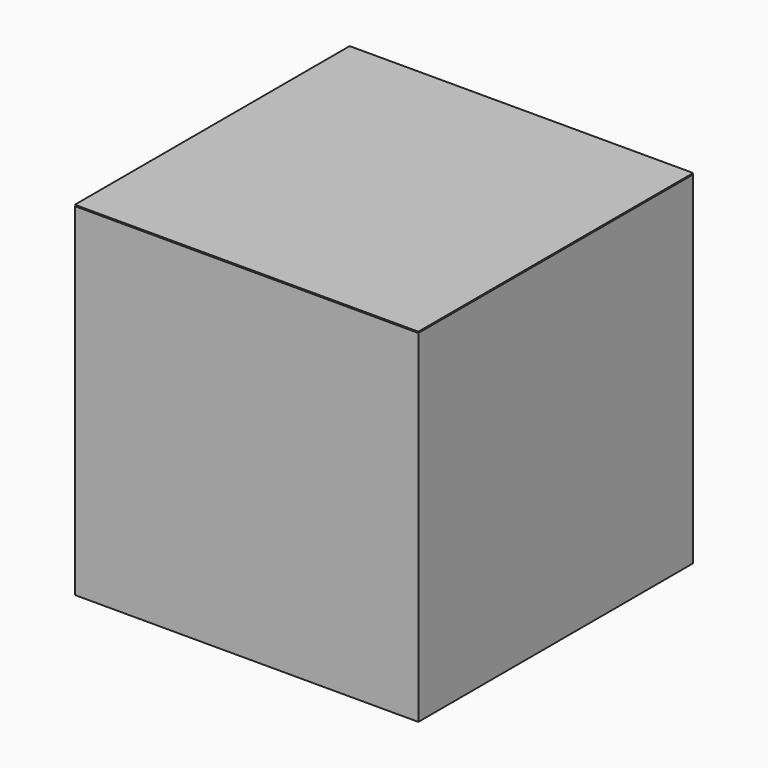
from build123d import *

# Parameters (mm, degrees)
F0_W         = 70
F0_H         = 70
F1_DEPTH     = 35
F2_T         = -3
F3_W         = 70
F3_H         = 70
F4_DEPTH     = 3
F5_SIZE      = 2.99999
F6_T1_DEPTH  = 64
F6_T3_DEPTH  = 64
F6_T9_DEPTH  = 72.3579697109
F6_T15_DEPTH = 72.3579697109
F6_T24_DEPTH = 72.3579697109
F6_T30_DEPTH = 72.3579697109
F6_T39_DEPTH = 72.3579697109
F6_T45_DEPTH = 72.3579697109
F6_T54_DEPTH = 72.3579697109
F6_T60_DEPTH = 72.3579697109


# Not quite as in the source:
# - a fillet or chamfer that OpenCascade refuses, or shapes differently, is made with other operations: its cross-section is extruded or revolved along the edge and cut away or added
# - a fillet or chamfer is up to 0.001 mm smaller than in the source, because OpenCascade refuses the exact size


with BuildPart() as f1:
    # F0 (on Top) → F1 (new body, symmetric)
    with BuildSketch(Plane.XY):
        Rectangle(F0_W, F0_H)
    extrude(amount=F1_DEPTH, both=True)

    # F2
    f2_openings = [f1.faces().sort_by_distance(p)[0] for p in [
        (0, 0, 35),
    ]]
    offset(amount=F2_T, openings=f2_openings)

    # F6: chamfer of 3.25 on 4 edges, made by hand

    # F6_s2 → F6_t1 (cut)
    with BuildSketch(Plane.YZ.offset(-32)):
        Polygon((-35.25, 35), (-32, 31.75), (-32, 35), align=None)
        Polygon((35.25, 35), (32, 31.75), (32, 35), align=None)
    extrude(amount=F6_T1_DEPTH, mode=Mode.SUBTRACT)

    # F6_s4 → F6_t3 (cut)
    with BuildSketch(Plane.XZ.offset(-32)):
        Polygon((-35.25, 35), (-32, 31.75), (-32, 35), align=None)
        Polygon((35.25, 35), (32, 31.75), (32, 35), align=None)
    extrude(amount=F6_T3_DEPTH, mode=Mode.SUBTRACT)


with BuildPart() as f4:
    # F3 (on face) → F4 (new body)
    with BuildSketch(Plane.XY.offset(35)):
        Rectangle(F3_W, F3_H)
    extrude(amount=-F4_DEPTH)

    # F5 (size 3 in the source; OpenCascade refuses exactly that, so slightly less here)
    f5_edges = [f4.edges().sort_by_distance(p)[0] for p in [
        (0, 35, 32),
        (-35, 0, 32),
        (0, -35, 32),
        (35, 0, 32),
    ]]
    chamfer(f5_edges, length=F5_SIZE)


with BuildPart() as f6_tool7:
    # F6_s8 → F6_t9 (new body)
    with BuildSketch(Plane.YZ.offset(-40.3579697109)):
        Polygon((-35.25, 35), (-32, 31.75), (-32, 35), align=None)
    extrude(amount=F6_T9_DEPTH)

    split(bisect_by=Plane.XZ.offset(35), keep=Keep.BOTTOM)

    split(bisect_by=Plane.YZ.offset(-35), keep=Keep.TOP)

    split(bisect_by=Plane.YZ.offset(-32), keep=Keep.BOTTOM)


with BuildPart() as f6_tool13:
    # F6_s14 → F6_t15 (new body)
    with BuildSketch(Plane.XZ.offset(-32)):
        Polygon((-35.25, 35), (-32, 31.75), (-32, 35), align=None)
    extrude(amount=F6_T15_DEPTH)

    split(bisect_by=Plane.XZ.offset(35), keep=Keep.BOTTOM)

    split(bisect_by=Plane.YZ.offset(-35), keep=Keep.TOP)

    split(bisect_by=Plane.XZ.offset(32), keep=Keep.TOP)


with BuildPart() as f6_tool7_1:
    add(f6_tool7.part)

    # F6_t19: intersect F6_tool13
    add(f6_tool13.part, mode=Mode.INTERSECT)


with BuildPart() as f1_1:
    add(f1.part)

    # F6_t5: cut F6_tool7
    add(f6_tool7_1.part, mode=Mode.SUBTRACT)


with BuildPart() as f6_tool22:
    # F6_s23 → F6_t24 (new body)
    with BuildSketch(Plane.YZ.offset(-32)):
        Polygon((-35.25, 35), (-32, 31.75), (-32, 35), align=None)
    extrude(amount=F6_T24_DEPTH)

    split(bisect_by=Plane.XZ.offset(35), keep=Keep.BOTTOM)

    split(bisect_by=Plane.YZ.offset(35), keep=Keep.BOTTOM)

    split(bisect_by=Plane.YZ.offset(32), keep=Keep.TOP)


with BuildPart() as f6_tool28:
    # F6_s29 → F6_t30 (new body)
    with BuildSketch(Plane.XZ.offset(40.3579697109)):
        Polygon((35.25, 35), (32, 31.75), (32, 35), align=None)
    extrude(amount=-F6_T30_DEPTH)

    split(bisect_by=Plane.XZ.offset(35), keep=Keep.BOTTOM)

    split(bisect_by=Plane.YZ.offset(35), keep=Keep.BOTTOM)

    split(bisect_by=Plane.XZ.offset(32), keep=Keep.TOP)


with BuildPart() as f6_tool22_1:
    add(f6_tool22.part)

    # F6_t34: intersect F6_tool28
    add(f6_tool28.part, mode=Mode.INTERSECT)


with BuildPart() as f1_2:
    add(f1_1.part)

    # F6_t20: cut F6_tool22
    add(f6_tool22_1.part, mode=Mode.SUBTRACT)


with BuildPart() as f6_tool37:
    # F6_s38 → F6_t39 (new body)
    with BuildSketch(Plane.XZ.offset(-40.3579697109)):
        Polygon((-35.25, 35), (-32, 31.75), (-32, 35), align=None)
    extrude(amount=F6_T39_DEPTH)

    split(bisect_by=Plane.YZ.offset(-35), keep=Keep.TOP)

    split(bisect_by=Plane.XZ.offset(-35), keep=Keep.TOP)

    split(bisect_by=Plane.XZ.offset(-32), keep=Keep.BOTTOM)


with BuildPart() as f6_tool43:
    # F6_s44 → F6_t45 (new body)
    with BuildSketch(Plane.YZ.offset(32)):
        Polygon((35.25, 35), (32, 31.75), (32, 35), align=None)
    extrude(amount=-F6_T45_DEPTH)

    split(bisect_by=Plane.YZ.offset(-35), keep=Keep.TOP)

    split(bisect_by=Plane.XZ.offset(-35), keep=Keep.TOP)

    split(bisect_by=Plane.YZ.offset(-32), keep=Keep.BOTTOM)


with BuildPart() as f6_tool37_1:
    add(f6_tool37.part)

    # F6_t49: intersect F6_tool43
    add(f6_tool43.part, mode=Mode.INTERSECT)


with BuildPart() as f1_3:
    add(f1_2.part)

    # F6_t35: cut F6_tool37
    add(f6_tool37_1.part, mode=Mode.SUBTRACT)


with BuildPart() as f6_tool52:
    # F6_s53 → F6_t54 (new body)
    with BuildSketch(Plane.YZ.offset(40.3579697109)):
        Polygon((35.25, 35), (32, 31.75), (32, 35), align=None)
    extrude(amount=-F6_T54_DEPTH)

    split(bisect_by=Plane.XZ.offset(-35), keep=Keep.TOP)

    split(bisect_by=Plane.YZ.offset(35), keep=Keep.BOTTOM)

    split(bisect_by=Plane.YZ.offset(32), keep=Keep.TOP)


with BuildPart() as f6_tool58:
    # F6_s59 → F6_t60 (new body)
    with BuildSketch(Plane.XZ.offset(32)):
        Polygon((35.25, 35), (32, 31.75), (32, 35), align=None)
    extrude(amount=-F6_T60_DEPTH)

    split(bisect_by=Plane.XZ.offset(-35), keep=Keep.TOP)

    split(bisect_by=Plane.YZ.offset(35), keep=Keep.BOTTOM)

    split(bisect_by=Plane.XZ.offset(-32), keep=Keep.BOTTOM)


with BuildPart() as f6_tool52_1:
    add(f6_tool52.part)

    # F6_t64: intersect F6_tool58
    add(f6_tool58.part, mode=Mode.INTERSECT)


with BuildPart() as f1_4:
    add(f1_3.part)

    # F6_t50: cut F6_tool52
    add(f6_tool52_1.part, mode=Mode.SUBTRACT)


solid = Compound([f4.part, f1_4.part])
